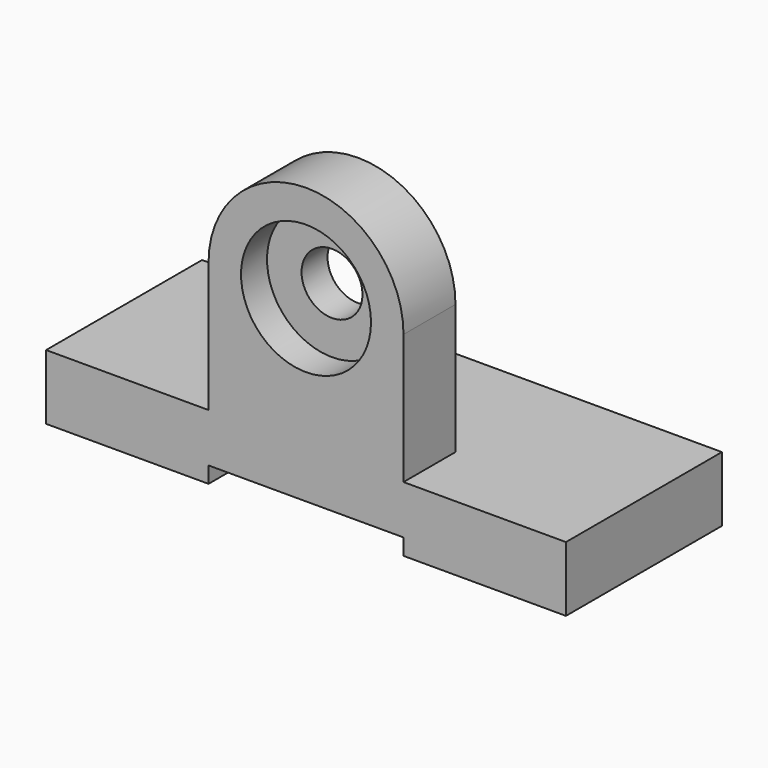
from build123d import *

# Parameters (mm, degrees)
F0_W           = 101.6
F0_H           = 38.1
F1_DEPTH       = 12.7
F3_DEPTH       = 12.7
F4_D           = 11.90625
F4_CBORE_D     = 25.4
F4_CBORE_DEPTH = 6.35
F5_W           = 38.1
F5_H           = 3.175
F6_DEPTH       = 38.101


# Not quite as in the source:
# - a length typed as a fraction of an inch, garbled in the dataset ("3 / 203.2 mm" for 3/8 in), is restored


with BuildPart() as f1:
    # F0 (on Top) → F1 (new body)
    with BuildSketch(Plane.XY):
        with Locations((50.8, 19.05)):
            Rectangle(F0_W, F0_H)
    extrude(amount=F1_DEPTH)

    # F2 (on face) → F3 (join)
    with BuildSketch(Plane.XZ):
        with BuildLine():
            Line((31.75, 38.1), (31.75, 0))
            Line((31.75, 0), (69.85, 0))
            Line((69.85, 0), (69.85, 38.1))
            ThreePointArc((69.85, 38.1), (50.8, 57.15), (31.75, 38.1))
        make_face()
    extrude(amount=-F3_DEPTH)

    # F4 (through all)
    with Locations(Plane.XZ):
        with Locations((50.8, 38.1)):
            CounterBoreHole(F4_D / 2, F4_CBORE_D / 2, F4_CBORE_DEPTH)

    # F5 (on face) → F6 (cut, through all)
    with BuildSketch(Plane(origin=(0, 38.1, 0), x_dir=(-1, 0, 0), z_dir=(0, 1, 0))):
        with Locations((-50.8, 1.5875)):
            Rectangle(F5_W, F5_H)
    extrude(amount=-F6_DEPTH, mode=Mode.SUBTRACT)


solid = f1.part
